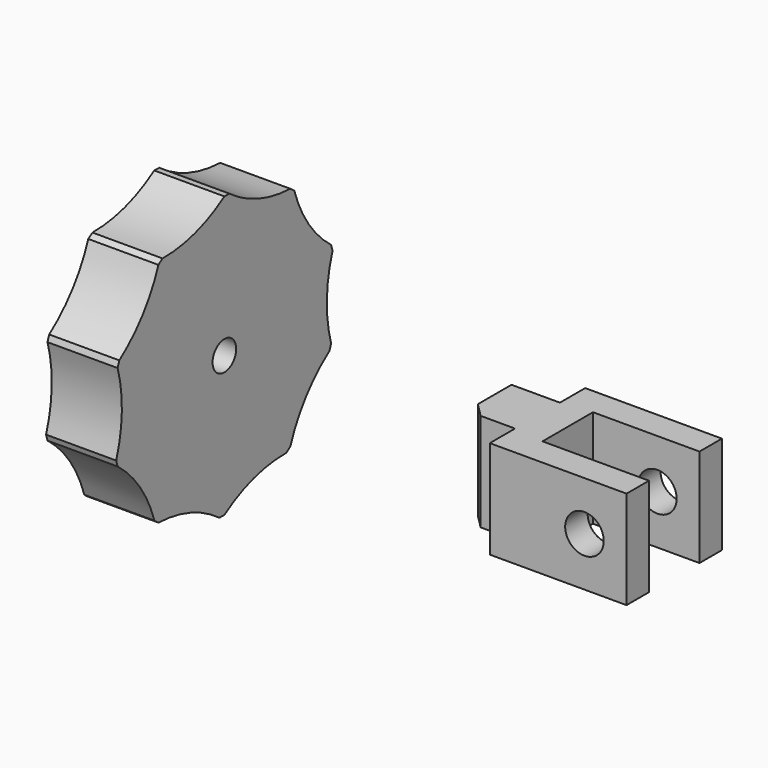
from build123d import *

# Parameters (mm, degrees)
F0_W        = 4.3133612332
F0_H        = 14
F0_W_2      = 15.1871098731
F0_R        = 2.75
F1_DEPTH    = 8.5
F2_DEPTH    = 4.5
F0_W_3      = 6.9083605352
F3_DEPTH    = 4
F5_R        = 2.1
F6_DEPTH    = 3.3
F7_DEPTH    = 7.3
F8_T1_DEPTH = 24.2867319519
F9_R        = 20
F9_R_2      = 2.1
F10_DEPTH   = 10
F11_DEPTH   = 5
F14_DEPTH   = 25


# Not quite as in the source:
# - a fillet or chamfer that OpenCascade refuses, or shapes differently, is made with other operations: its cross-section is extruded or revolved along the edge and cut away or added
# - a feature names something its author has since deleted; it is built from what else it names


with BuildPart() as f1:
    # F0 (on Front) → F1 (new body, symmetric)
    with BuildSketch(Plane.XZ):
        with Locations((56.8073878317, 43.8252027185)):
            Rectangle(F0_W, F0_H)
        with Locations((66.5576233848, 43.8252027185)):
            Rectangle(F0_W_2, F0_H)
        with Locations((68.1511783214, 43.8252027185)):
            Circle(F0_R, mode=Mode.SUBTRACT)
    extrude(amount=F1_DEPTH, both=True)

    # F0 (on Front) → F2 (cut, symmetric)
    with BuildSketch(Plane.XZ):
        with Locations((66.5576233848, 43.8252027185)):
            Rectangle(F0_W_2, F0_H)
        with Locations((68.1511783214, 43.8252027185)):
            Circle(F0_R, mode=Mode.SUBTRACT)
    extrude(amount=F2_DEPTH, both=True, mode=Mode.SUBTRACT)

    # F0 (on Front) → F3 (join, symmetric)
    with BuildSketch(Plane.XZ):
        with Locations((51.1965269475, 43.8252027185)):
            Rectangle(F0_W_3, F0_H)
    extrude(amount=F3_DEPTH, both=True)

    # F5 (on offset) → F6 (cut)
    with BuildSketch(Plane(origin=(54.7423466799, 0, 0), x_dir=(0, -1, 0), z_dir=(-1, 0, 0))):
        Polygon((2.0207259422, 47.3252027185), (-2.0207259422, 47.3252027185), (-4, 47.3252027185), (-4, 40.3252027185), (2.0207259422, 40.3252027185), (4.0414518843, 43.8252027185), align=None)
        with Locations((0, 43.8252027185)):
            Circle(F5_R, mode=Mode.SUBTRACT)
    extrude(amount=F6_DEPTH, mode=Mode.SUBTRACT)

    # F5 (on offset) → F7 (cut, symmetric)
    with BuildSketch(Plane(origin=(54.7423466799, 0, 0), x_dir=(0, -1, 0), z_dir=(-1, 0, 0))):
        with Locations((0, 43.8252027185)):
            Circle(F5_R)
    extrude(amount=F7_DEPTH, both=True, mode=Mode.SUBTRACT)

    # F8: chamfer of 2 on 1 edges, made by hand

    # F8_s2 → F8_t1 (cut)
    with BuildSketch(Plane.XY.offset(31.6818367426)):
        Polygon((47.7423466799, -2), (49.7423466799, -4), (47.7423466799, -4), align=None)
    extrude(amount=F8_T1_DEPTH, mode=Mode.SUBTRACT)


with BuildPart() as f10:
    # F9 (on Right) → F10 (new body)
    with BuildSketch(Plane.YZ):
        with Locations((0, 43.8252027185)):
            Circle(F9_R)
        Polygon((-4.1569219382, 43.8252027185), (-2.0784609691, 47.4252027185), (2.0784609691, 47.4252027185), (4.1569219382, 43.8252027185), (2.0784609691, 40.2252027185), (-2.0784609691, 40.2252027185), align=None, mode=Mode.SUBTRACT)
        Polygon((2.0784609691, 47.4252027185), (-2.0784609691, 47.4252027185), (-4.1569219382, 43.8252027185), (-2.0784609691, 40.2252027185), (2.0784609691, 40.2252027185), (4.1569219382, 43.8252027185), align=None)
        with Locations((0, 43.8252027185)):
            Circle(F9_R_2, mode=Mode.SUBTRACT)
    extrude(amount=F10_DEPTH)

    # F9 (on Right) → F11 (cut)
    with BuildSketch(Plane.YZ):
        Polygon((2.0784609691, 47.4252027185), (-2.0784609691, 47.4252027185), (-4.1569219382, 43.8252027185), (-2.0784609691, 40.2252027185), (2.0784609691, 40.2252027185), (4.1569219382, 43.8252027185), align=None)
        with Locations((0, 43.8252027185)):
            Circle(F9_R_2, mode=Mode.SUBTRACT)
    extrude(amount=F11_DEPTH, mode=Mode.SUBTRACT)

    # F13 (on face) → F14 (cut)
    with BuildSketch(Plane.YZ.offset(10)):
        with BuildLine():
            ThreePointArc((12.4671096682, 59.4639742981), (15.0235182276, 54.2354326614), (19.0211303259, 50.005542606))
            ThreePointArc((19.0211303259, 50.005542606), (16.4390631424, 55.2163046406), (12.4671096682, 59.4639742981))
        make_face()
        with BuildLine():
            ThreePointArc((0.8938642938, 63.8052178993), (6.035301928, 61.0778581094), (11.7557050458, 60.005542606))
            ThreePointArc((11.7557050458, 60.005542606), (6.6039597367, 62.7034366347), (0.8938642938, 63.8052178993))
        make_face()
        with BuildLine():
            ThreePointArc((-11.0208068595, 60.5147747971), (-5.2581945757, 61.3303555942), (0, 63.8252027185))
            ThreePointArc((0, 63.8252027185), (-5.7536318282, 62.9797249205), (-11.0208068595, 60.5147747971))
        make_face()
        with BuildLine():
            ThreePointArc((-18.7259043759, 50.8494824186), (-14.5432394709, 54.8964796588), (-11.7557050458, 60.005542606))
            ThreePointArc((-11.7557050458, 60.005542606), (-15.9135315934, 55.9396367633), (-18.7259043759, 50.8494824186))
        make_face()
        with BuildLine():
            ThreePointArc((-19.2783428908, 38.5011539411), (-18.2732611948, 44.233752231), (-19.0211303259, 50.005542606))
            ThreePointArc((-19.0211303259, 50.005542606), (-19.995003171, 44.2722465555), (-19.2783428908, 38.5011539411))
        make_face()
        with BuildLine():
            ThreePointArc((-19.0211303259, 37.644862831), (-16.4390631424, 32.4341007964), (-12.4671096682, 28.1864311388))
            ThreePointArc((-12.4671096682, 28.1864311388), (-15.0235182276, 33.4149727756), (-19.0211303259, 37.644862831))
        make_face()
        with BuildLine():
            ThreePointArc((-11.7557050458, 27.644862831), (-6.6039597367, 24.9469688022), (-0.8938642938, 23.8451875377))
            ThreePointArc((-0.8938642938, 23.8451875377), (-6.035301928, 26.5725473276), (-11.7557050458, 27.644862831))
        make_face()
        with BuildLine():
            ThreePointArc((0, 23.8252027185), (5.7536318282, 24.6706805165), (11.0208068595, 27.1356306399))
            ThreePointArc((11.0208068595, 27.1356306399), (5.2581945757, 26.3200498428), (0, 23.8252027185))
        make_face()
        with BuildLine():
            ThreePointArc((11.7557050458, 27.644862831), (15.9135315934, 31.7107686737), (18.7259043759, 36.8009230184))
            ThreePointArc((18.7259043759, 36.8009230184), (14.5432394709, 32.7539257782), (11.7557050458, 27.644862831))
        make_face()
        with BuildLine():
            ThreePointArc((19.0211303259, 37.644862831), (19.7537668119, 40.6965134177), (20, 43.8252027185))
            ThreePointArc((20, 43.8252027185), (19.8187645656, 46.5115703575), (19.2783428908, 49.1492514959))
            ThreePointArc((19.2783428908, 49.1492514959), (18.2732611948, 43.4166532059), (19.0211303259, 37.644862831))
        make_face()
    extrude(amount=-F14_DEPTH, mode=Mode.SUBTRACT)


solid = Compound([f1.part, f10.part])
